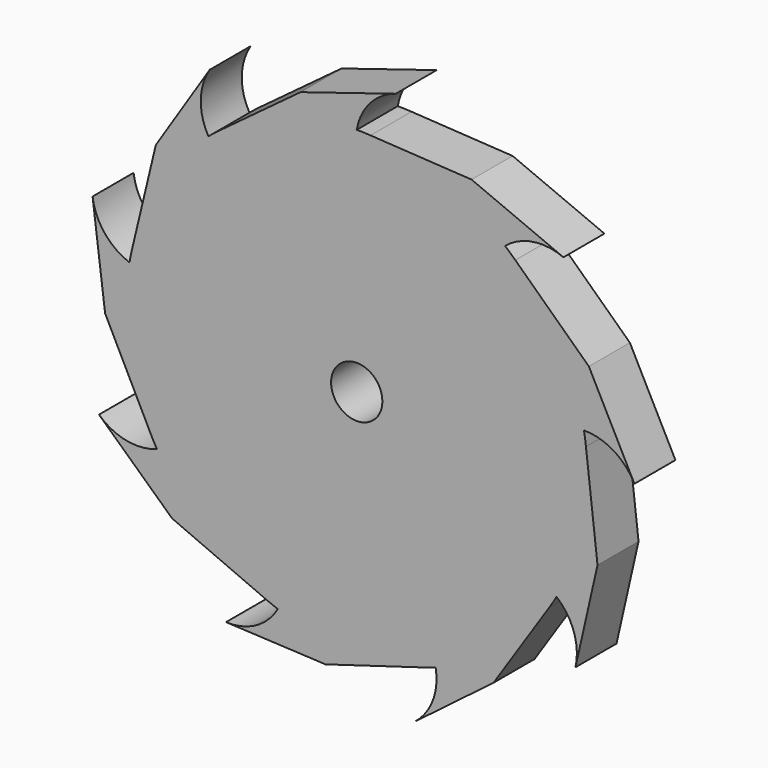
from build123d import *

# Parameters (mm, degrees)
F0_R     = 2.5
F1_DEPTH = 5


# Not quite as in the source:
# - a feature names something its author has since deleted; it is built from what else it names


with BuildPart() as f1:
    # F0 (on Front) → F1 (new body)
    with BuildSketch(Plane.XZ):
        with BuildLine():
            ThreePointArc((19.4855715851, -11.25), (21.7333310915, -5.8234285148), (22.5, 0))
            ThreePointArc((22.5, 0), (22.4630219271, 1.2894362728), (22.3522092532, 2.5746342462))
            ThreePointArc((22.3522092532, 2.5746342462), (22.2651615708, 3.2423109389), (22.1581744428, 3.9070839975))
            ThreePointArc((22.1581744428, 3.9070839975), (19.8134723767, 10.6619094152), (15.4678426969, 16.3400074145))
            ThreePointArc((15.4678426969, 16.3400074145), (14.9719859982, 16.795524263), (14.4627212179, 17.2359999702))
            ThreePointArc((14.4627212179, 17.2359999702), (8.3246571453, 20.9033510092), (1.3459006368, 22.4597095145))
            ThreePointArc((1.3459006368, 22.4597095145), (0.6732517819, 22.489925123), (0, 22.5))
            ThreePointArc((0, 22.5), (-7.0593576826, 21.363882351), (-13.4058032893, 18.0702639208))
            ThreePointArc((-13.4058032893, 18.0702639208), (-13.9405044255, 17.6610400702), (-14.4627212179, 17.2359999702))
            ThreePointArc((-14.4627212179, 17.2359999702), (-19.1402205948, 11.8280157078), (-21.8847828674, 5.22554101))
            ThreePointArc((-21.8847828674, 5.22554101), (-22.0313436808, 4.568358088), (-22.1581744428, 3.9070839975))
            ThreePointArc((-22.1581744428, 3.9070839975), (-22.2651615708, -3.2423109389), (-20.1236293196, -10.0642706148))
            ThreePointArc((-20.1236293196, -10.0642706148), (-19.8134723767, -10.6619094152), (-19.4855715851, -11.25))
            ThreePointArc((-19.4855715851, -11.25), (-14.9719859982, -16.795524263), (-8.9464059639, -20.6448981671))
            ThreePointArc((-8.9464059639, -20.6448981671), (-8.3246571453, -20.9033510092), (-7.6954532248, -21.1430839677))
            ThreePointArc((-7.6954532248, -21.1430839677), (-0.6732517819, -22.489925123), (6.4169401705, -21.5655484245))
            ThreePointArc((6.4169401705, -21.5655484245), (7.0593576826, -21.363882351), (7.6954532248, -21.1430839677))
            ThreePointArc((7.6954532248, -21.1430839677), (13.9405044255, -17.6610400702), (18.7777286828, -12.3954388997))
            ThreePointArc((18.7777286828, -12.3954388997), (19.1402205948, -11.8280157078), (19.4855715851, -11.25))
        make_face()
        Circle(F0_R, mode=Mode.SUBTRACT)
        with BuildLine():
            ThreePointArc((-13.4058032893, 18.0702639208), (-7.0593576826, 21.363882351), (0, 22.5))
            ThreePointArc((0, 22.5), (1.2893242582, 25.1998179584), (3.7992770591, 26.8281640483))
            Line((3.7992770591, 26.8281640483), (-5.477073051, 23.9523583039))
            Line((-5.477073051, 23.9523583039), (-13.4058032893, 18.0702639208))
        make_face()
        with BuildLine():
            ThreePointArc((-21.8847828674, 5.22554101), (-19.1402205948, 11.8280157078), (-14.4627212179, 17.2359999702))
            ThreePointArc((-14.4627212179, 17.2359999702), (-15.2104510666, 20.1329421727), (-14.3343963619, 22.9936942077))
            Line((-14.3343963619, 22.9936942077), (-19.5919605158, 14.8279762838))
            Line((-19.5919605158, 14.8279762838), (-21.8847828674, 5.22554101))
        make_face()
        with BuildLine():
            Line((-24.5395519148, -1.2345806341), (-20.1236293196, -10.0642706148))
            ThreePointArc((-20.1236293196, -10.0642706148), (-22.2651615708, -3.2423109389), (-22.1581744428, 3.9070839975))
            ThreePointArc((-22.1581744428, 3.9070839975), (-24.5930872921, 5.6456389916), (-25.7608464161, 8.4002193008))
            Line((-25.7608464161, 8.4002193008), (-24.5395519148, -1.2345806341))
        make_face()
        with BuildLine():
            Line((-18.0048142462, -16.7194635525), (-8.9464059639, -20.6448981671))
            ThreePointArc((-8.9464059639, -20.6448981671), (-14.9719859982, -16.795524263), (-19.4855715851, -11.25))
            ThreePointArc((-19.4855715851, -11.25), (-22.4683446518, -11.4833214179), (-25.1335101323, -10.1238115749))
            Line((-25.1335101323, -10.1238115749), (-18.0048142462, -16.7194635525))
        make_face()
        with BuildLine():
            Line((-3.0454238906, -24.3811236585), (6.4169401705, -21.5655484245))
            ThreePointArc((6.4169401705, -21.5655484245), (-0.6732517819, -22.489925123), (-7.6954532248, -21.1430839677))
            ThreePointArc((-7.6954532248, -21.1430839677), (-9.8304138412, -23.2391081131), (-12.7459251298, -23.9107985011))
            Line((-12.7459251298, -23.9107985011), (-3.0454238906, -24.3811236585))
        make_face()
        with BuildLine():
            ThreePointArc((22.3522092532, 2.5746342462), (22.4630219271, 1.2894362728), (22.5, 0))
            ThreePointArc((22.5, 0), (21.7333310915, -5.8234285148), (19.4855715851, -11.25))
            ThreePointArc((19.4855715851, -11.25), (21.1790203936, -13.7164965405), (21.3342330732, -16.7043524734))
            Line((21.3342330732, -16.7043524734), (23.4818872972, -7.2328947514))
            Line((23.4818872972, -7.2328947514), (22.3522092532, 2.5746342462))
        make_face()
        with BuildLine():
            Line((13.3389541496, -20.6345850387), (18.7777286828, -12.3954388997))
            ThreePointArc((18.7777286828, -12.3954388997), (13.9405044255, -17.6610400702), (7.6954532248, -21.1430839677))
            ThreePointArc((7.6954532248, -21.1430839677), (7.4072768587, -24.1210578483), (5.6056198962, -26.5096570697))
            Line((5.6056198962, -26.5096570697), (13.3389541496, -20.6345850387))
        make_face()
        with BuildLine():
            ThreePointArc((1.3459006368, 22.4597095145), (8.3246571453, 20.9033510092), (14.4627212179, 17.2359999702))
            ThreePointArc((14.4627212179, 17.2359999702), (17.1858104334, 18.4754188566), (20.1552265199, 18.1094377689))
            Line((20.1552265199, 18.1094377689), (11.2005977653, 21.8691656728))
            Line((11.2005977653, 21.8691656728), (1.3459006368, 22.4597095145))
        make_face()
        with BuildLine():
            ThreePointArc((15.4678426969, 16.3400074145), (19.8134723767, 10.6619094152), (22.1581744428, 3.9070839975))
            ThreePointArc((22.1581744428, 3.9070839975), (25.0408649078, 3.1061659404), (27.0803214916, 0.9171042935))
            Line((27.0803214916, 0.9171042935), (22.6373844064, 9.5531473747))
            Line((22.6373844064, 9.5531473747), (15.4678426969, 16.3400074145))
        make_face()
    extrude(amount=F1_DEPTH)


solid = f1.part
